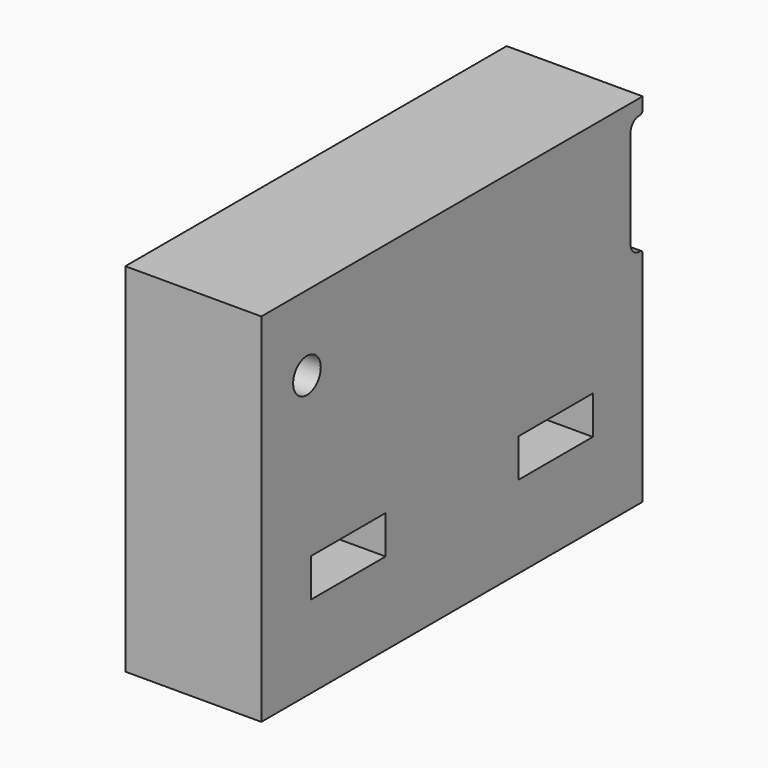
from build123d import *

# Parameters (mm, degrees)
F0_W      = 41
F0_H      = 11
F0_R      = 1.5875
F0_R_2    = 1.75
F1_DEPTH  = 10
F2_DEPTH  = 12.5
F3_R      = 1
F4_DEPTH  = 14
F5_SIZE   = 0.5
F6_DEPTH  = 19
F7_R      = 2.2
F8_DEPTH  = 20
F9_W      = 8.55
F9_H      = 3.5222247243
F10_DEPTH = 22.3


with BuildPart() as f1:
    # F0 (on Right) → F1 (new body)
    with BuildSketch(Plane.YZ):
        Rectangle(F0_W, F0_H)
        with Locations((-16.6625, 0)):
            Circle(F0_R, mode=Mode.SUBTRACT)
        with Locations((-4.475, 0)):
            Circle(F0_R_2, mode=Mode.SUBTRACT)
    extrude(amount=-F1_DEPTH)

    # F0 (on Right) → F2 (join)
    with BuildSketch(Plane.YZ):
        with BuildLine():
            Line((-20.5, 5.5), (20.5, 5.5))
            Line((20.5, 5.5), (21.5708505204, 5.5))
            ThreePointArc((21.5708505204, 5.5), (21.8035943853, 5.5964056654), (21.9000000507, 5.8291495303))
            Line((21.9000000507, 5.8291495303), (21.9000000507, 6.9000000507))
            Line((21.9000000507, 6.9000000507), (-21.9000000507, 6.9000000507))
            Line((-21.9000000507, 6.9000000507), (-21.9000000507, -6.9000000507))
            Line((-21.9000000507, -6.9000000507), (21.9000000507, -6.9000000507))
            Line((21.9000000507, -6.9000000507), (21.9000000507, -5.8291495303))
            ThreePointArc((21.9000000507, -5.8291495303), (21.8035943853, -5.5964056654), (21.5708505204, -5.5))
            Line((21.5708505204, -5.5), (20.5, -5.5))
            Line((20.5, -5.5), (-20.5, -5.5))
            Line((-20.5, -5.5), (-20.5, 5.5))
        make_face()
    extrude(amount=-F2_DEPTH)

    # F3
    f3_edges = [f1.edges().sort_by_distance(p)[0] for p in [
        (-10, 0, 5.5),
        (-10, -20.5, 0),
        (-10, 0, -5.5),
        (-10, 20.5, 0),
        (-5, 20.5, -5.5),
        (-5, 20.5, 5.5),
    ]]
    fillet(f3_edges, radius=F3_R)

    # F0 (on Right) → F4 (join)
    with BuildSketch(Plane.YZ):
        with Locations((-4.475, 0)):
            Circle(F0_R_2)
    extrude(amount=-F4_DEPTH)

    # F5
    f5_edges = [f1.edges().sort_by_distance(p)[0] for p in [
        (-14, -6.225, 0),
    ]]
    chamfer(f5_edges, length=F5_SIZE)

    # F6 (add): a face of the model
    f6_faces = [f1.faces().sort_by_distance(p)[0] for p in [
        (-6.25, 0, -6.9000000507),
    ]]
    extrude(f6_faces, amount=F6_DEPTH)

    # F7 (on face) → F8 (cut)
    with BuildSketch(Plane(origin=(0, 0, -25.9000000507), x_dir=(1, 0, 0), z_dir=(0, 0, -1))):
        with Locations((-6.1999997124, 11.8999998271)):
            Circle(F7_R)
        with Locations((-6.1999997124, -11.9000002742)):
            Circle(F7_R)
    extrude(amount=-F8_DEPTH, mode=Mode.SUBTRACT)

    # F9 (on face) → F10 (cut)
    with BuildSketch(Plane(origin=(-12.5, 0, 0), x_dir=(0, -1, 0), z_dir=(-1, 0, 0))):
        with Locations((-11.9000004627, -16.5611151606)):
            Rectangle(F9_W, F9_H)
        with Locations((11.9000000857, -16.5611151606)):
            Rectangle(F9_W, F9_H)
    extrude(amount=-F10_DEPTH, mode=Mode.SUBTRACT)


solid = f1.part
